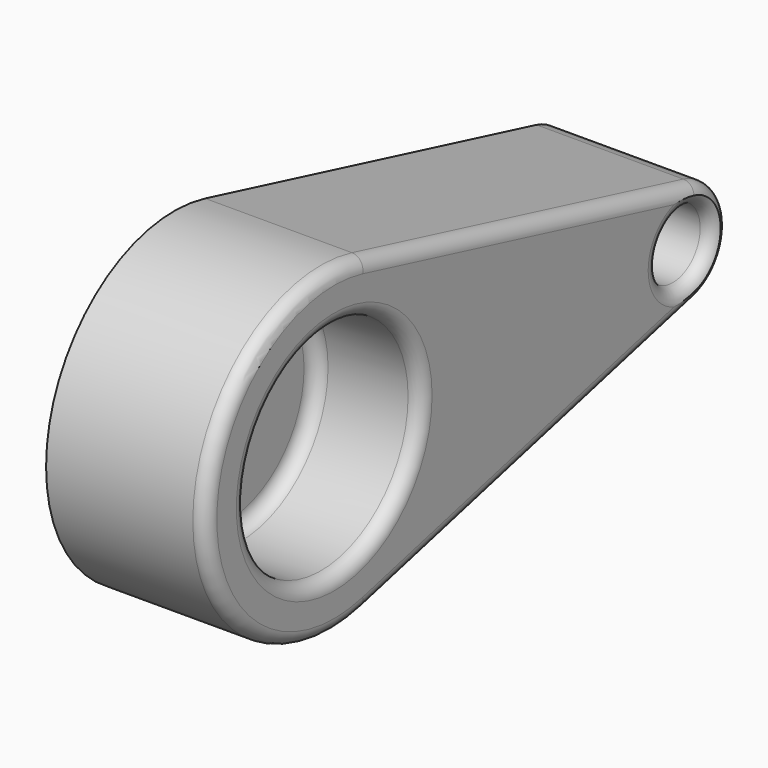
from build123d import *

# Parameters (mm, degrees)
F1_DEPTH     = 76.2
F2_R         = 51.8976641698
F2_R_2       = 16.2693021543
F3_DEPTH     = 50.8
F4_T5_DEPTH  = 203.2
F4_T7_DEPTH  = 203.2
F4_T10_ANGLE = 208.0724869359
F4_T12_ANGLE = 151.9275130641
F5_T         = -2.54


# Not quite as in the source:
# - a fillet or chamfer that OpenCascade refuses, or shapes differently, is made with other operations: its cross-section is extruded or revolved along the edge and cut away or added


with BuildPart() as f1:
    # F0 (on Right) → F1 (new body)
    with BuildSketch(Plane.YZ):
        with BuildLine():
            ThreePointArc((18.4812146278, -73.9248585111), (60.0612543768, -46.8944103565), (76.2, 0))
            ThreePointArc((76.2, 0), (60.0612543768, 46.8944103565), (18.4812146278, 73.9248585111))
            ThreePointArc((18.4812146278, 73.9248585111), (-76.2, 0), (18.4812146278, -73.9248585111))
        make_face()
        with BuildLine():
            ThreePointArc((18.4812146278, 73.9248585111), (60.0612543768, 46.8944103565), (76.2, 0))
            ThreePointArc((76.2, 0), (60.0612543768, -46.8944103565), (18.4812146278, -73.9248585111))
            Line((18.4812146278, -73.9248585111), (215.6141706573, -24.6416195037))
            ThreePointArc((215.6141706573, -24.6416195037), (184.0537657814, 0), (215.6141706573, 24.6416195037))
            Line((215.6141706573, 24.6416195037), (18.4812146278, 73.9248585111))
        make_face()
        with BuildLine():
            ThreePointArc((234.8537657814, 0), (229.474183907, 15.6314701188), (215.6141706573, 24.6416195037))
            ThreePointArc((215.6141706573, 24.6416195037), (184.0537657814, 0), (215.6141706573, -24.6416195037))
            ThreePointArc((215.6141706573, -24.6416195037), (229.474183907, -15.6314701188), (234.8537657814, 0))
        make_face()
    extrude(amount=F1_DEPTH)

    # F2 (on face) → F3 (cut)
    with BuildSketch(Plane.YZ.offset(76.2)):
        Circle(F2_R)
        with Locations((209.4537657814, 0)):
            Circle(F2_R_2)
    extrude(amount=-F3_DEPTH, mode=Mode.SUBTRACT)

    # F4: fillet of radius 6.35 on 8 edges, made by hand

    # F4_s1 → F4_t2 (revolve)
    with BuildSketch(Plane.XY):
        with BuildLine():
            ThreePointArc((31.75, 51.8976641698), (27.2598719395, 50.0377922304), (25.4, 45.5476641698))
            Line((25.4, 45.5476641698), (25.4, 51.8976641698))
            Line((25.4, 51.8976641698), (31.75, 51.8976641698))
        make_face()
    revolve(axis=Axis((25.4, 0, 0), (1, 0, 0)))

    # F4_s3 → F4_t4 (revolve)
    with BuildSketch(Plane.XY):
        with BuildLine():
            ThreePointArc((31.75, 225.7230679357), (27.2598719395, 223.8631959962), (25.4, 219.3730679357))
            Line((25.4, 219.3730679357), (25.4, 225.7230679357))
            Line((25.4, 225.7230679357), (31.75, 225.7230679357))
        make_face()
    revolve(axis=Axis((25.4, 209.4537657814, 0), (1, 0, 0)))

    # F4_s6 → F4_t5 (cut)
    with BuildSketch(Plane(origin=(0, 197.1329560295, -49.2832390074), x_dir=(1, 0, 0), z_dir=(0, -0.9701425001, 0.242535625))):
        with BuildLine():
            ThreePointArc((69.85, 76.2), (74.3401280605, 74.3401280605), (76.2, 69.85))
            Line((76.2, 69.85), (76.2, 76.2))
            Line((76.2, 76.2), (69.85, 76.2))
        make_face()
    extrude(amount=F4_T5_DEPTH, mode=Mode.SUBTRACT)

    # F4_s8 → F4_t7 (cut)
    with BuildSketch(Plane(origin=(0, 0, 0), x_dir=(1, 0, 0), z_dir=(0, 0.9701425001, 0.242535625))):
        with BuildLine():
            ThreePointArc((69.85, 76.2), (74.3401280605, 74.3401280605), (76.2, 69.85))
            Line((76.2, 69.85), (76.2, 76.2))
            Line((76.2, 76.2), (69.85, 76.2))
        make_face()
    extrude(amount=F4_T7_DEPTH, mode=Mode.SUBTRACT)

    # F4_s9 → F4_t10 (revolve, cut)
    with BuildSketch(Plane(origin=(0, 0, 0), x_dir=(1, 0, 0), z_dir=(0, 0.9701425001, -0.242535625))):
        with BuildLine():
            ThreePointArc((69.85, -76.2), (74.3401280605, -74.3401280605), (76.2, -69.85))
            Line((76.2, -69.85), (76.2, -76.2))
            Line((76.2, -76.2), (69.85, -76.2))
        make_face()
    revolve(axis=Axis((76.2, 0, 0), (1, 0, 0)), revolution_arc=F4_T10_ANGLE, mode=Mode.SUBTRACT)

    # F4_s11 → F4_t12 (revolve, cut)
    with BuildSketch(Plane(origin=(0, 197.1329560295, 49.2832390074), x_dir=(1, 0, 0), z_dir=(0, -0.9701425001, -0.242535625))):
        with BuildLine():
            ThreePointArc((76.2, -69.85), (74.3401280605, -74.3401280605), (69.85, -76.2))
            Line((69.85, -76.2), (76.2, -76.2))
            Line((76.2, -76.2), (76.2, -69.85))
        make_face()
    revolve(axis=Axis((76.2, 209.4537657814, 0), (1, 0, 0)), revolution_arc=F4_T12_ANGLE, mode=Mode.SUBTRACT)

    # F4_s13 → F4_t14 (revolve, cut)
    with BuildSketch(Plane.XY):
        with BuildLine():
            ThreePointArc((76.2, 58.2476641698), (74.3401280605, 53.7575361093), (69.85, 51.8976641698))
            Line((69.85, 51.8976641698), (76.2, 51.8976641698))
            Line((76.2, 51.8976641698), (76.2, 58.2476641698))
        make_face()
    revolve(axis=Axis((76.2, 0, 0), (1, 0, 0)), mode=Mode.SUBTRACT)

    # F4_s15 → F4_t16 (revolve, cut)
    with BuildSketch(Plane.XY):
        with BuildLine():
            ThreePointArc((76.2, 232.0730679357), (74.3401280605, 227.5829398752), (69.85, 225.7230679357))
            Line((69.85, 225.7230679357), (76.2, 225.7230679357))
            Line((76.2, 225.7230679357), (76.2, 232.0730679357))
        make_face()
    revolve(axis=Axis((76.2, 209.4537657814, 0), (1, 0, 0)), mode=Mode.SUBTRACT)

    # F5
    f5_openings = [f1.faces().sort_by_distance(p)[0] for p in [
        (0, 57.51924, 0),
    ]]
    offset(amount=F5_T, openings=f5_openings)


solid = f1.part
